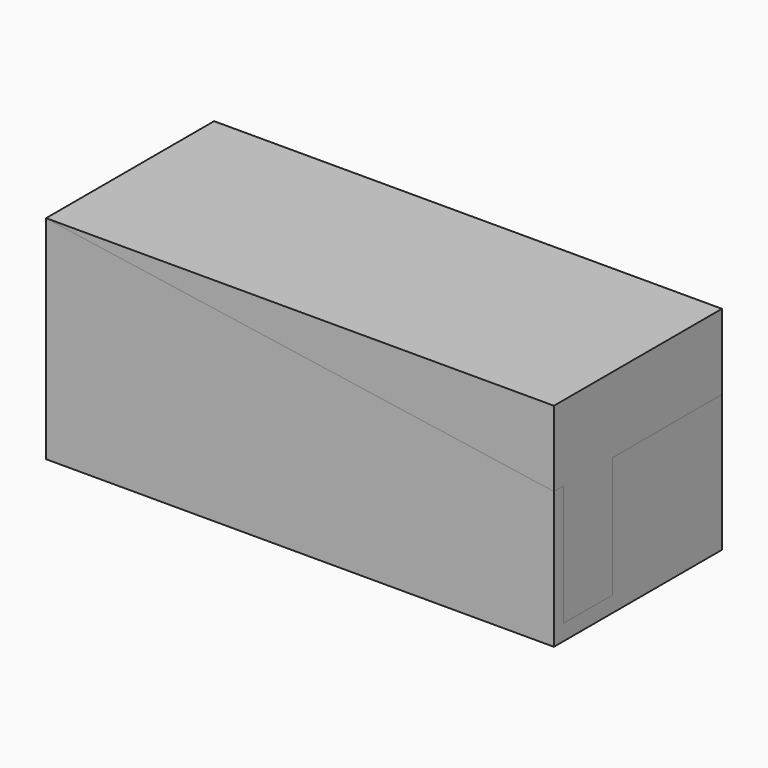
from build123d import *

# Parameters (mm, degrees)
F0_W     = 60.4586862028
F0_H     = 25.266315788
F1_DEPTH = 25
F2_W     = 25
F2_H     = 16.2828955799
F3_W     = 25
F3_H     = 25.266315788
F6_DEPTH = 1
F7_W     = 7.3107741773
F7_H     = 20.593938767
F8_DEPTH = 13.20027


with BuildPart() as f1:
    # F0 (on Front) → F1 (new body)
    with BuildSketch(Plane.XZ):
        with Locations((-30.2293431014, 12.633157894)):
            Rectangle(F0_W, F0_H)
    extrude(amount=F1_DEPTH)


with BuildPart() as f4:
    # F2 (on face) → F4 section 0
    with BuildSketch(Plane.YZ):
        with Locations((-12.5, 8.14144779)):
            Rectangle(F2_W, F2_H)
    # F3 (on face) → F4 section 1
    with BuildSketch(Plane(origin=(-60.4586862028, 0, 0), x_dir=(0, -1, 0), z_dir=(-1, 0, 0))):
        with Locations((12.5, 12.633157894)):
            Rectangle(F3_W, F3_H)
    loft()

    # F5 (on face) → F6 (cut, symmetric)
    with BuildSketch(Plane(origin=(2.3671755739, 0, 15.9311622853), x_dir=(0.9891403353, 0, -0.1469741378), z_dir=(0.1469741378, 0, 0.9891403353))):
        with BuildLine():
            Line((-2.3931645385, -3.5427620169), (-52.2132776678, -3.5427620169))
            ThreePointArc((-52.2132776678, -3.5427620169), (-61.4906333919, -11.2389497301), (-51.5840724111, -18.1063134223))
            Line((-51.5840724111, -18.1063134223), (-15.5934300274, -18.1063134223))
            Line((-15.5934300274, -18.1063134223), (-15.5934300274, -16.1147173494))
            Line((-15.5934300274, -16.1147173494), (-2.3931645385, -16.1147173494))
            Line((-2.3931645385, -16.1147173494), (-2.3931645385, -3.5427620169))
        make_face()
    extrude(amount=F6_DEPTH, both=True, mode=Mode.SUBTRACT)

    # F7 (on Right) → F8 (cut)
    with BuildSketch(Plane.YZ):
        with Locations((-19.9142117053, 12.1830397402)):
            Rectangle(F7_W, F7_H)
    extrude(amount=-F8_DEPTH, mode=Mode.SUBTRACT)


solid = Compound([f1.part, f4.part])
